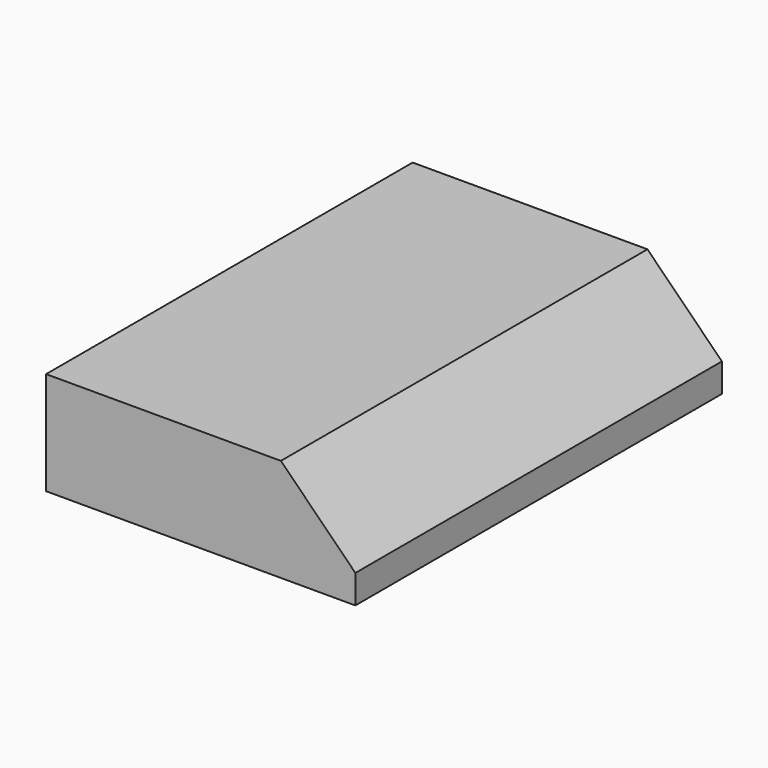
from build123d import *

# Parameters (mm, degrees)
F1_DEPTH = 400


# Not quite as in the source:
# - a feature names something its author has since deleted; it is built from what else it names


with BuildPart() as f1:
    # F0 (on Front) → F1 (new body)
    with BuildSketch(Plane.XZ):
        Polygon((-270, 0), (0, 0), (0, 25), (-65, 90), (-270, 90), align=None)
    extrude(amount=F1_DEPTH)


solid = f1.part
